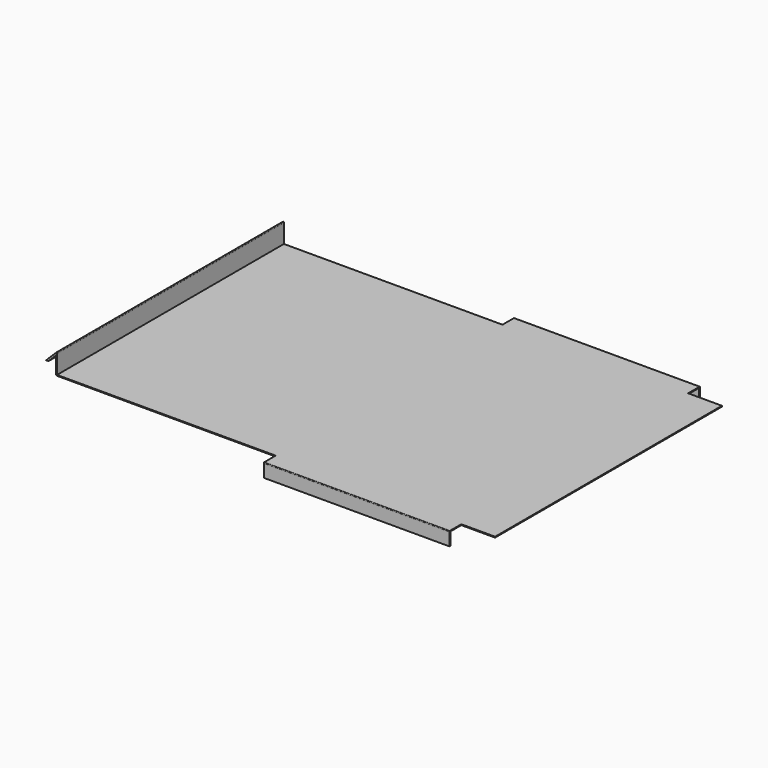
from build123d import *

# Parameters (mm, degrees)
F1_DEPTH  = 1.25
F2_W      = 275
F2_H      = 2
F3_DEPTH  = 20
F4_W      = 1.25
F4_H      = 420
F5_DEPTH  = 30
F6_W      = 420
F6_H      = 15
F7_DEPTH  = 15
F8_SIZE   = 14.99999
F10_R     = 1
F11_R     = 1
F12_DEPTH = 442.001


# Not quite as in the source:
# - a fillet or chamfer is up to 0.001 mm smaller than in the source, because OpenCascade refuses the exact size


with BuildPart() as f1:
    # F0 (on Top) → F1 (new body)
    with BuildSketch(Plane.XY):
        Polygon((0, -232), (275, -232), (275, -210), (325, -210), (325, 210), (275, 210), (275, 232), (0, 232), (0, 210), (-325, 210), (-325, -210), (0, -210), align=None)
    extrude(amount=F1_DEPTH)

    # F2 (on face) → F3 (join)
    with BuildSketch(Plane.XY.offset(1.25)):
        with Locations((137.5, 231)):
            Rectangle(F2_W, F2_H)
        with Locations((137.5, -231)):
            Rectangle(F2_W, F2_H)
    extrude(amount=-F3_DEPTH)

    # F4 (on face) → F5 (join)
    with BuildSketch(Plane(origin=(0, 0, 0), x_dir=(1, 0, 0), z_dir=(0, 0, -1))):
        with Locations((-324.375, 0)):
            Rectangle(F4_W, F4_H)
    extrude(amount=-F5_DEPTH)

    # F6 (on face) → F7 (join)
    with BuildSketch(Plane(origin=(-325, 0, 0), x_dir=(0, -1, 0), z_dir=(-1, 0, 0))):
        with Locations((0, 22.5)):
            Rectangle(F6_W, F6_H)
    extrude(amount=F7_DEPTH)

    # F8 (size 15 in the source; OpenCascade refuses exactly that, so slightly less here)
    f8_edges = [f1.edges().sort_by_distance(p)[0] for p in [
        (-340, 0, 30),
    ]]
    chamfer(f8_edges, length=F8_SIZE)

    # F10
    f10_edges = [f1.edges().sort_by_distance(p)[0] for p in [
        (-323.75, 0, 30),
    ]]
    fillet(f10_edges, radius=F10_R)

    # F11
    f11_edges = [f1.edges().sort_by_distance(p)[0] for p in [
        (-325, 0, 0),
        (137.5, 232, 1.25),
        (137.5, -232, 1.25),
    ]]
    fillet(f11_edges, radius=F11_R)

    # F9 (on face) → F12 (cut, through all)
    with BuildSketch(Plane(origin=(0, 210, 0), x_dir=(-1, 0, 0), z_dir=(0, 1, 0))):
        Polygon((336.4644660941, 15), (325, 26.4644660941), (325, 15), align=None)
    extrude(amount=-F12_DEPTH, mode=Mode.SUBTRACT)


solid = f1.part
